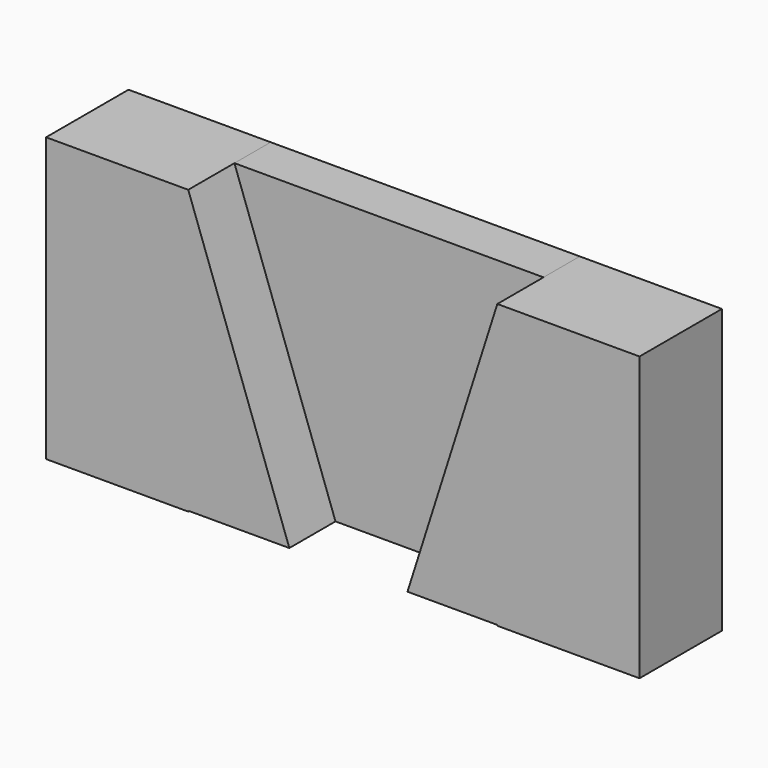
from build123d import *

# Parameters (mm, degrees)
F1_DEPTH = 25.4
F3_DEPTH = 11.176


# Not quite as in the source:
# - a feature of the source that left no trace in its solid (it failed there, or was rolled back) is left out


with BuildPart() as f1:
    # F0 (on Front) → F1 (new body)
    with BuildSketch(Plane.XZ):
        Polygon((-10.2070893071, 38.031912598), (-45.2590893071, 38.031912598), (-45.2590893071, -31.818087402), (-10.2070893071, -31.818087402), (-10.2070893071, -31.6261931479), (14.7131280974, -31.6261931479), align=None)
    extrude(amount=F1_DEPTH)


with BuildPart() as f1b:
    # F0 (on Front) → F1, piece 2 (new body)
    with BuildSketch(Plane.XZ):
        Polygon((101.0449106929, 38.031912598), (65.9929106929, 38.031912598), (43.8374243677, -31.6261931479), (65.9929106929, -31.6261931479), (65.9929106929, -31.818087402), (101.0449106929, -31.818087402), align=None)
    extrude(amount=F1_DEPTH)


with BuildPart() as f3:
    # F0 (on Front) → F3 (new body)
    with BuildSketch(Plane.XZ):
        Polygon((65.9929106929, 38.031912598), (-10.2070893071, 38.031912598), (14.7131280974, -31.6261931479), (43.8374243677, -31.6261931479), align=None)
    extrude(amount=F3_DEPTH)


solid = Compound([f1.part, f1b.part, f3.part])
